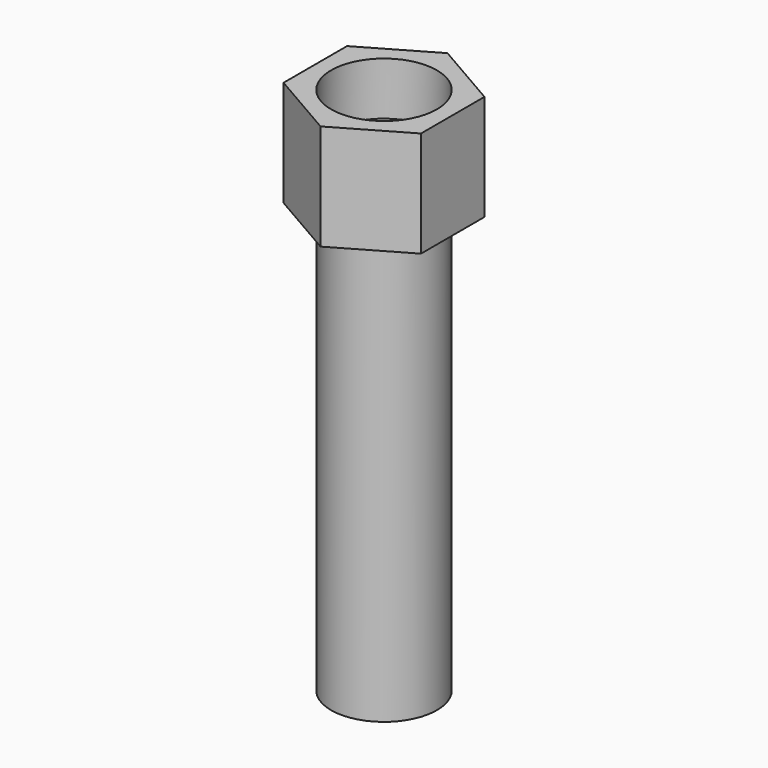
from build123d import *

# Parameters (mm, degrees)
F0_W     = 0.25
F0_H     = 2
F2_R     = 0.25
F3_DEPTH = 0.5
F4_R     = 0.25
F5_DEPTH = 0.25


# Not quite as in the source:
# - a pattern or mirror of a feature is missing from the dataset's text; its kind, count and spacing are read off the source's solid


with BuildPart() as f1:
    # F0 (on Front) → F1 (revolve)
    with BuildSketch(Plane.XZ):
        with Locations((-0.125, 1)):
            Rectangle(F0_W, F0_H)
    revolve(axis=Axis((0, 0, 1), (0, 0, 1)))

    # F1_copies: F1 across plane


with BuildPart() as f1_1:
    add(f1.part)
    add(f1.part.mirror(Plane.XY.offset(1.125)))

    # F2 (on face) → F3 (join)
    with BuildSketch(Plane.XY.offset(2)):
        Polygon((0.3247595264, 0.1875), (0, 0.375), (-0.3247595264, 0.1875), (-0.3247595264, -0.1875), (0, -0.375), (0.3247595264, -0.1875), align=None)
        Circle(F2_R, mode=Mode.SUBTRACT)
    extrude(amount=F3_DEPTH)

    # F4 (on face) → F5 (cut)
    with BuildSketch(Plane.XY.offset(2.5)):
        Circle(F4_R)
    extrude(amount=-F5_DEPTH, mode=Mode.SUBTRACT)


solid = f1_1.part
